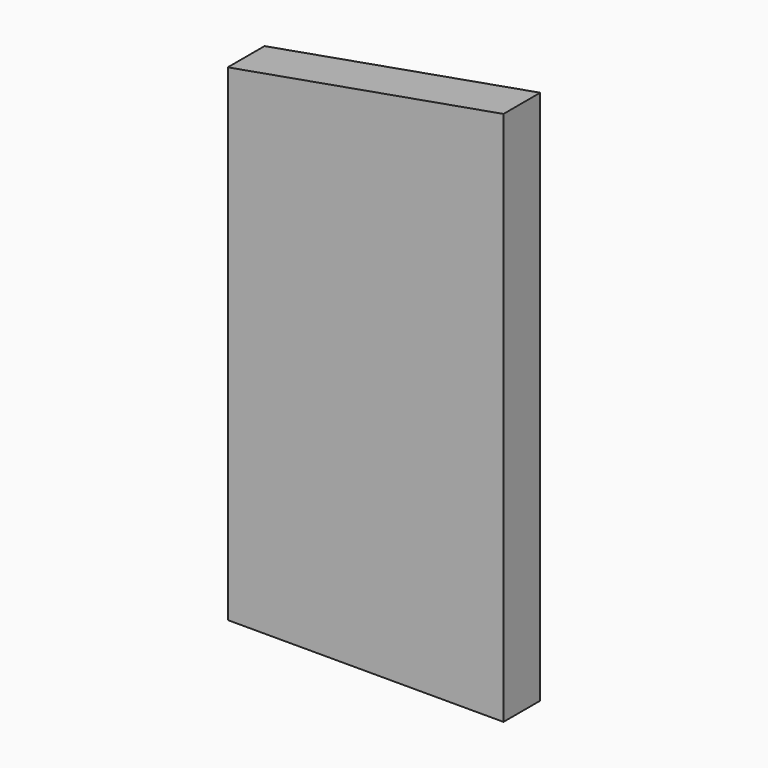
from build123d import *

# Parameters (mm, degrees)
F0_W        = 152.4
F0_H        = 304.8
F1_DEPTH    = 25.4
F2_T1_DEPTH = 1081.4461668656


# Not quite as in the source:
# - a fillet or chamfer that OpenCascade refuses, or shapes differently, is made with other operations: its cross-section is extruded or revolved along the edge and cut away or added


with BuildPart() as f1:
    # F0 (on Front) → F1 (new body)
    with BuildSketch(Plane.XZ):
        with Locations((-29.3548897063, -4.3910965323)):
            Rectangle(F0_W, F0_H)
    extrude(amount=F1_DEPTH)

    # F2: chamfer of 203.2 x 35.82964248 on 1 edges, made by hand

    # F2_s2 → F2_t1 (cut)
    with BuildSketch(Plane.XZ.offset(-528.0230834328)):
        Polygon((97.6451102937, 148.0089034677), (-105.5548897063, 112.1792609877), (-105.5548897063, 148.0089034677), align=None)
    extrude(amount=F2_T1_DEPTH, mode=Mode.SUBTRACT)


solid = f1.part
